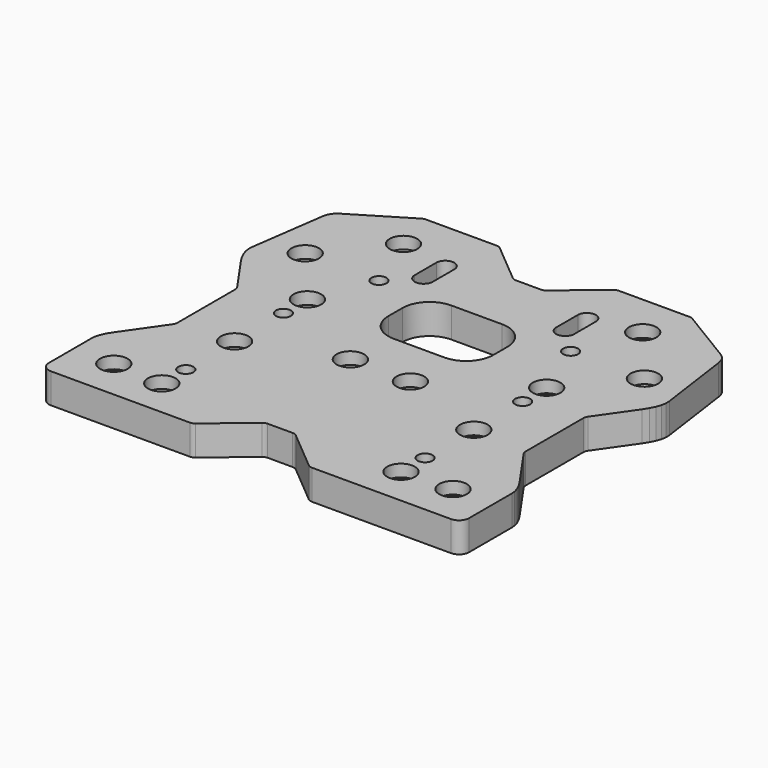
from build123d import *

# Parameters (mm, degrees)
F0_R     = 4.6
F0_R_2   = 2.5
F1_DEPTH = 10
F0_R_3   = 3.6
F2_DEPTH = 6


# Not quite as in the source:
# - ends of sketch curves that miss each other by under 0.0002 mm in the source are joined


with BuildPart() as f1:
    # F0 (on Top) → F1 (new body)
    with BuildSketch(Plane.XY):
        with BuildLine():
            Line((-45.12993, 63.520274), (-63.589038, 52.344512))
            Line((-63.589038, 52.344512), (-64.491972, 51.645644))
            Line((-64.491972, 51.645644), (-65.195294, 50.763356))
            Line((-65.195294, 50.763356), (-65.706925, 49.675321))
            Line((-65.706925, 49.675321), (-66.018102, 48.35028))
            Line((-66.018102, 48.35028), (-69.517849, 23.448285))
            Line((-69.517849, 23.448285), (-69.565467, 22.06741))
            Line((-69.565467, 22.06741), (-69.321375, 20.551373))
            Line((-69.321375, 20.551373), (-68.771557, 18.920731))
            Line((-68.771557, 18.920731), (-67.92238, 17.202201))
            Line((-67.92238, 17.202201), (-66.786009, 15.407932))
            Line((-66.786009, 15.407932), (-58.427898, 3.420306))
            ThreePointArc((-58.427898, 3.420306), (-58.1136589115, 2.780672761), (-58.0056, 2.076258))
            Line((-58.0056, 2.076258), (-58.0056, -21.994915))
            ThreePointArc((-58.0056, -21.994915), (-58.1134934985, -22.6988030848), (-58.427266754, -23.3380571713))
            Line((-58.427266754, -23.3380571713), (-67.733177, -36.698447))
            Line((-67.733177, -36.698447), (-68.737483, -38.320327))
            Line((-68.737483, -38.320327), (-69.450198, -39.883875))
            Line((-69.450198, -39.883875), (-69.867581, -41.370908))
            Line((-69.867581, -41.370908), (-70, -42.7495))
            Line((-70, -42.7495), (-70, -60.5007))
            ThreePointArc((-70, -60.5007), (-69.01608381, -62.87608381), (-66.6407, -63.86))
            Line((-66.6407, -63.86), (-20.34613, -63.86))
            ThreePointArc((-20.34613, -63.86), (-19.5423824877, -63.718277595), (-18.8355788311, -63.3102042013))
            Line((-18.8355788311, -63.3102042013), (-5.655221, -52.25057))
            ThreePointArc((-5.655221, -52.25057), (-4.9484172103, -51.8424972951), (-4.14467, -51.700775))
            Line((-4.14467, -51.700775), (4.14467, -51.700775))
            ThreePointArc((4.14467, -51.700775), (4.9484172103, -51.8424972951), (5.6552206765, -52.2505703856))
            Line((5.6552206765, -52.2505703856), (18.835579, -63.310204))
            ThreePointArc((18.835579, -63.310204), (19.5423824877, -63.718277595), (20.34613, -63.86))
            Line((20.34613, -63.86), (66.64, -63.86))
            ThreePointArc((66.64, -63.86), (69.0158787848, -62.8758787848), (70, -60.5))
            Line((70, -60.5), (70, -42.7495))
            Line((70, -42.7495), (69.867655, -41.370921))
            Line((69.867655, -41.370921), (69.45051, -39.883911))
            Line((69.45051, -39.883911), (68.738189, -38.320362))
            Line((68.738189, -38.320362), (67.734411, -36.698447))
            Line((67.734411, -36.698447), (58.431323, -23.33483))
            ThreePointArc((58.431323, -23.33483), (58.1178034861, -22.6957823028), (58.01, -21.992181))
            Line((58.01, -21.992181), (58.01, 2.079652))
            ThreePointArc((58.01, 2.079652), (58.1179688317, 2.7837800001), (58.4319542472, 3.4232068277))
            Line((58.4319542472, 3.4232068277), (66.783488, 15.407932))
            Line((66.783488, 15.407932), (67.921136, 17.204755))
            Line((67.921136, 17.204755), (68.770985, 18.924136))
            Line((68.770985, 18.924136), (69.321132, 20.553655))
            Line((69.321132, 20.553655), (69.565833, 22.06785))
            Line((69.565833, 22.06785), (69.51871, 23.448285))
            Line((69.51871, 23.448285), (66.018963, 48.35028))
            Line((66.018963, 48.35028), (65.698808, 49.700863))
            Line((65.698808, 49.700863), (65.172247, 50.800958))
            Line((65.172247, 50.800958), (64.474805, 51.662632))
            Line((64.474805, 51.662632), (63.589037, 52.344512))
            Line((63.589037, 52.344512), (45.129929, 63.520274))
            ThreePointArc((45.129929, 63.520274), (44.5446477821, 63.7734755253), (43.912842, 63.86))
            Line((43.912842, 63.86), (20.34613, 63.86))
            ThreePointArc((20.34613, 63.86), (19.5423827897, 63.7182777049), (18.8355793235, 63.3102046144))
            Line((18.8355793235, 63.3102046144), (5.655221, 52.250571))
            ThreePointArc((5.655221, 52.250571), (4.9484175123, 51.842497405), (4.14467, 51.700775))
            Line((4.14467, 51.700775), (-4.14467, 51.700775))
            ThreePointArc((-4.14467, 51.700775), (-4.9484175123, 51.842497405), (-5.6552211689, 52.2505707987))
            Line((-5.6552211689, 52.2505707987), (-18.835579, 63.310205))
            ThreePointArc((-18.835579, 63.310205), (-19.5423827897, 63.7182777049), (-20.34613, 63.86))
            Line((-20.34613, 63.86), (-43.912843, 63.86))
            ThreePointArc((-43.912843, 63.86), (-44.5446487821, 63.7734755253), (-45.12993, 63.520274))
        make_face()
        with Locations((-56.5, -50.34)):
            Circle(F0_R, mode=Mode.SUBTRACT)
        with Locations((-39.85, -51.178)):
            Circle(F0_R, mode=Mode.SUBTRACT)
        with Locations((-39.85, -41.178)):
            Circle(F0_R_2, mode=Mode.SUBTRACT)
        with Locations((-39.85, -20.858)):
            Circle(F0_R, mode=Mode.SUBTRACT)
        with Locations((-39.85, -0.538)):
            Circle(F0_R_2, mode=Mode.SUBTRACT)
        with Locations((-10, -9.96)):
            Circle(F0_R, mode=Mode.SUBTRACT)
        with Locations((39.85, -51.178)):
            Circle(F0_R, mode=Mode.SUBTRACT)
        with Locations((56.5, -50.34)):
            Circle(F0_R, mode=Mode.SUBTRACT)
        with Locations((39.85, -41.178)):
            Circle(F0_R_2, mode=Mode.SUBTRACT)
        with Locations((10, -9.96)):
            Circle(F0_R, mode=Mode.SUBTRACT)
        with Locations((39.85, -20.858)):
            Circle(F0_R, mode=Mode.SUBTRACT)
        with Locations((39.85, -0.538)):
            Circle(F0_R_2, mode=Mode.SUBTRACT)
        with Locations((-39.85, 9.462)):
            Circle(F0_R, mode=Mode.SUBTRACT)
        with Locations((-56.5, 29.36)):
            Circle(F0_R, mode=Mode.SUBTRACT)
        with Locations((-31.925, 29.36)):
            Circle(F0_R_2, mode=Mode.SUBTRACT)
        with Locations((-39.85, 49.462)):
            Circle(F0_R, mode=Mode.SUBTRACT)
        with BuildLine():
            Line((-26.57, 37.54), (-26.57, 46.54))
            ThreePointArc((-26.57, 46.54), (-23.57, 49.54), (-20.57, 46.54))
            Line((-20.57, 46.54), (-20.57, 37.54))
            ThreePointArc((-20.57, 37.54), (-23.57, 34.54), (-26.57, 37.54))
        make_face(mode=Mode.SUBTRACT)
        with BuildLine():
            Line((-17.5, 15.199075), (-17.5, 21.099375))
            ThreePointArc((-17.5, 21.099375), (-14.8493603037, 27.4985853037), (-8.45015, 30.149225))
            Line((-8.45015, 30.149225), (8.45015, 30.149225))
            ThreePointArc((8.45015, 30.149225), (14.8493603037, 27.4985853037), (17.5, 21.099375))
            Line((17.5, 21.099375), (17.5, 15.199075))
            ThreePointArc((17.5, 15.199075), (14.8493603037, 8.7998646963), (8.45015, 6.149225))
            Line((8.45015, 6.149225), (-8.45015, 6.149225))
            ThreePointArc((-8.45015, 6.149225), (-14.8493603037, 8.7998646963), (-17.5, 15.199075))
        make_face(mode=Mode.SUBTRACT)
        with Locations((31.925, 29.36)):
            Circle(F0_R_2, mode=Mode.SUBTRACT)
        with Locations((39.85, 9.462)):
            Circle(F0_R, mode=Mode.SUBTRACT)
        with Locations((56.5, 29.36)):
            Circle(F0_R, mode=Mode.SUBTRACT)
        with BuildLine():
            Line((20.57, 37.54), (20.57, 46.54))
            ThreePointArc((20.57, 46.54), (23.57, 49.54), (26.57, 46.54))
            Line((26.57, 46.54), (26.57, 37.54))
            ThreePointArc((26.57, 37.54), (23.57, 34.54), (20.57, 37.54))
        make_face(mode=Mode.SUBTRACT)
        with Locations((39.85, 49.462)):
            Circle(F0_R, mode=Mode.SUBTRACT)
    extrude(amount=F1_DEPTH)

    # F0 (on Top) → F2 (join)
    with BuildSketch(Plane.XY):
        with Locations((-39.85, 9.462)):
            Circle(F0_R)
        with Locations((-39.85, 9.462)):
            Circle(F0_R_2, mode=Mode.SUBTRACT)
        with Locations((-39.85, -20.858)):
            Circle(F0_R)
        with Locations((-39.85, -20.858)):
            Circle(F0_R_2, mode=Mode.SUBTRACT)
        with Locations((-39.85, -51.178)):
            Circle(F0_R)
        with Locations((-39.85, -51.178)):
            Circle(F0_R_2, mode=Mode.SUBTRACT)
        with Locations((39.85, -20.858)):
            Circle(F0_R)
        with Locations((39.85, -20.858)):
            Circle(F0_R_3, mode=Mode.SUBTRACT)
        with Locations((39.85, -51.178)):
            Circle(F0_R)
        with Locations((39.85, -51.178)):
            Circle(F0_R_3, mode=Mode.SUBTRACT)
        with Locations((39.85, 9.462)):
            Circle(F0_R)
        with Locations((39.85, 9.462)):
            Circle(F0_R_3, mode=Mode.SUBTRACT)
        with Locations((-39.85, 49.462)):
            Circle(F0_R)
        with Locations((-39.85, 49.462)):
            Circle(F0_R_2, mode=Mode.SUBTRACT)
        with Locations((39.85, 49.462)):
            Circle(F0_R)
        with Locations((39.85, 49.462)):
            Circle(F0_R_3, mode=Mode.SUBTRACT)
        with Locations((-10, -9.96)):
            Circle(F0_R)
        with Locations((-10, -9.96)):
            Circle(F0_R_2, mode=Mode.SUBTRACT)
        with Locations((10, -9.96)):
            Circle(F0_R)
        with Locations((10, -9.96)):
            Circle(F0_R_2, mode=Mode.SUBTRACT)
        with Locations((-56.5, -50.34)):
            Circle(F0_R)
        with Locations((-56.5, -50.34)):
            Circle(F0_R_3, mode=Mode.SUBTRACT)
        with Locations((56.5, 29.36)):
            Circle(F0_R)
        with Locations((56.5, 29.36)):
            Circle(F0_R_2, mode=Mode.SUBTRACT)
        with Locations((56.5, -50.34)):
            Circle(F0_R)
        with Locations((56.5, -50.34)):
            Circle(F0_R_3, mode=Mode.SUBTRACT)
        with Locations((-56.5, 29.36)):
            Circle(F0_R)
        with Locations((-56.5, 29.36)):
            Circle(F0_R_2, mode=Mode.SUBTRACT)
    extrude(amount=F2_DEPTH)


solid = f1.part
